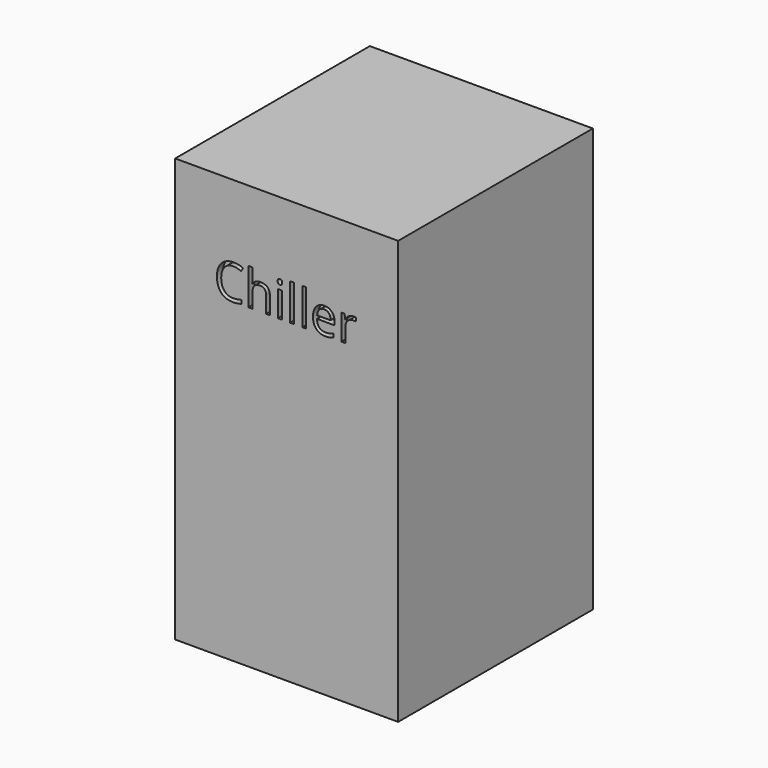
from build123d import *

# Parameters (mm, degrees)
F0_W         = 779.78
F0_H         = 850.9
F1_DEPTH     = 1480.82
F2_TEXT_SIZE = 168.0119890445
F3_DEPTH     = 25.4


# Not quite as in the source:
# - Text() gives the source's letters only with a copy of the font that has no kerning and outlines rounded to 1/6400 em; it was checked with that copy


with BuildPart() as f1:
    # F0 (on Top) → F1 (new body)
    with BuildSketch(Plane.XY):
        Rectangle(F0_W, F0_H)
    extrude(amount=F1_DEPTH)

    # F2 (on face) → F3 (cut)
    with BuildSketch(Plane.XZ.offset(425.45)):
        with Locations((-254, 1105.851367888)):
            Text('Chiller', F2_TEXT_SIZE, font='Open Sans', text_align=(TextAlign.LEFT, TextAlign.BOTTOM))
    extrude(amount=-F3_DEPTH, mode=Mode.SUBTRACT)


solid = f1.part
